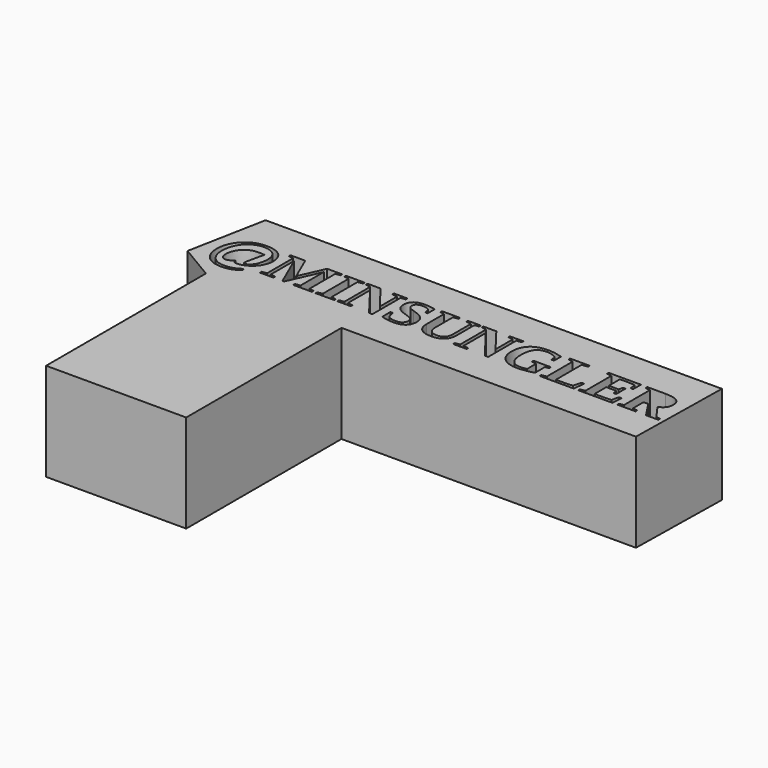
from build123d import *

# Parameters (mm, degrees)
F1_DEPTH     = 15
F2_TEXT_SIZE = 16.3802333797
F3_DEPTH     = 101.6
F4_DEPTH     = 12.7


# Not quite as in the source:
# - Text() gives the source's letters only with a copy of the font that has no kerning and outlines rounded to 1/6400 em; it was checked with that copy


with BuildPart() as f1:
    # F0 (on Top) → F1 (new body)
    with BuildSketch(Plane.XY):
        Polygon((75.721360743, 19.0308541059), (76.2574374676, 48.7833172083), (-52.9379397631, 48.7833172083), (-57.2265833616, 26.5359804034), (-47.3090969026, 20.6390954554), (-47.3090969026, -35.9173864126), (-7.6391454786, -35.9173864126), (-7.6391454786, 19.0308541059), align=None)
    extrude(amount=F1_DEPTH)

    # F2 (on face) → F3 (cut)
    with BuildSketch(Plane.XY.offset(15)):
        with Locations((-53.7133403122, 28.4122619778)):
            Text('@MINSUNGLER', F2_TEXT_SIZE, font='Tinos', font_style=FontStyle.BOLD, text_align=(TextAlign.LEFT, TextAlign.BOTTOM))
    extrude(amount=-F3_DEPTH, mode=Mode.SUBTRACT)

    # F4 (add): a face of the model
    f4_faces = [f1.faces().sort_by_distance(p)[0] for p in [
        (74.4087637219, 33.9355653778, 15),
    ]]
    extrude(f4_faces, amount=F4_DEPTH)


solid = f1.part
